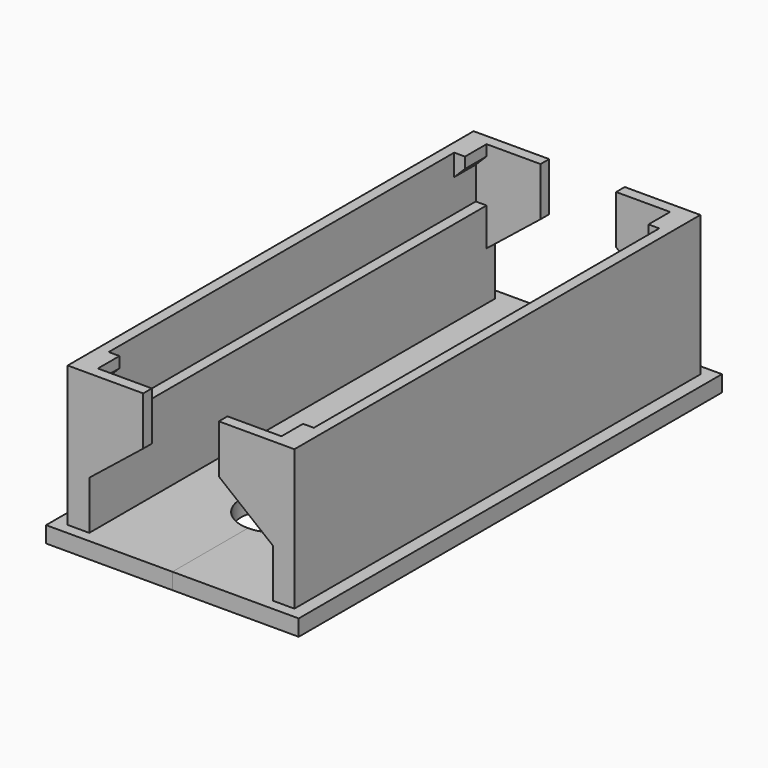
from build123d import *
from build123d import SkipClean  # not in build123d's __all__

# Parameters (mm, degrees)
F1_DEPTH = 1.5
F2_W     = 2
F2_H     = 23.5
F3_DEPTH = 8
F4_W     = 1
F4_H     = 23.5
F5_DEPTH = 5
F7_DEPTH = 1
F9_DEPTH = 2.5


# Not quite as in the source:
# - a feature names something its author has since deleted; it is built from what else it names


with BuildPart() as f1:
    # F0 (on Top) → F1 (new body)
    with BuildSketch(Plane.XY):
        with BuildLine():
            ThreePointArc((0, 9.25), (-3.25, 12.5), (0, 15.75))
            Line((0, 15.75), (0, 24.5))
            Line((0, 24.5), (-11.7, 24.5))
            Line((-11.7, 24.5), (-11.7, 0))
            Line((-11.7, 0), (0, 0))
            Line((0, 0), (0, 9.25))
        make_face()
    extrude(amount=F1_DEPTH)

    # F2 (on face) → F3 (join)
    with BuildSketch(Plane.XY.offset(1.5)):
        with Locations((-9.5, 11.75)):
            Rectangle(F2_W, F2_H)
    extrude(amount=F3_DEPTH)

    # F4 (on face) → F5 (join)
    with BuildSketch(Plane.XY.offset(9.5)):
        with Locations((-10, 11.75)):
            Rectangle(F4_W, F4_H)
    extrude(amount=F5_DEPTH)

    # F6 (on face) → F7 (join)
    with BuildSketch(Plane(origin=(0, 23.5, 0), x_dir=(-1, 0, 0), z_dir=(0, 1, 0))):
        Polygon((9.5, 9.5), (9.5, 14.5), (3.5, 14.5), (3.5, 10), (8.5, 6), (8.5, 9.5), align=None)
    extrude(amount=-F7_DEPTH)

    # F8 (on face) → F9 (join)
    with BuildSketch(Plane.XZ.offset(-22.5)):
        Polygon((-8.5, 14.5), (-9.5, 14.5), (-9.5, 12.5), (-8.5, 13.5), align=None)
    extrude(amount=F9_DEPTH)

    # F10: F1 across plane


with BuildPart() as f1_1:
    add(f1.part, clean=False)
    add(f1.part.mirror(Plane.XZ), clean=False)

    # F11: F1 across plane


with BuildPart() as f1_2:
    add(f1_1.part, clean=False)
    with SkipClean():  # cleaning this boolean's faces spoils the solid; the shape is the same uncleaned
        add(f1_1.part.mirror(Plane.YZ), clean=False)


solid = f1_2.part
